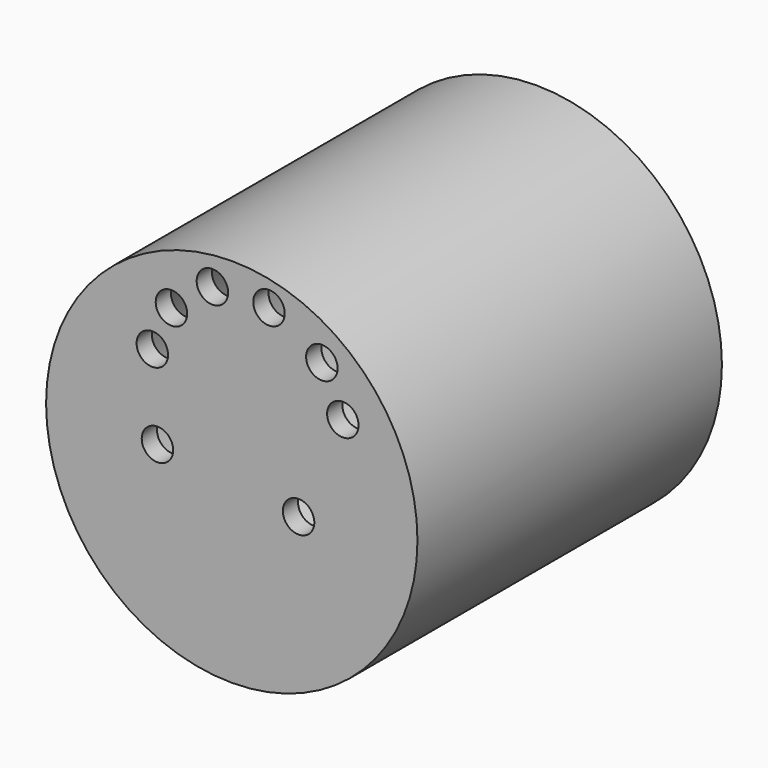
from build123d import *

# Parameters (mm, degrees)
F0_R     = 24.7867182939
F1_DEPTH = 50.8
F2_T     = -2.54
F7_D     = 4.2


# Not quite as in the source:
# - a feature of the source that left no trace in its solid (it failed there, or was rolled back) is left out


with BuildPart() as f1:
    # F0 (on Front) → F1 (new body)
    with BuildSketch(Plane.XZ):
        Circle(F0_R)
    extrude(amount=F1_DEPTH)

    # F2
    f2_openings = [f1.faces().sort_by_distance(p)[0] for p in [
        (0, 0, 0),
    ]]
    offset(amount=F2_T, openings=f2_openings)

    # F7 (through all)
    with Locations(Plane(origin=(0, 0, 0), x_dir=(1, 0, 0), z_dir=(0, 1, 0))):
        with Locations((8.9164366946, 2.3716597352), (14.8237738758, -10.9670488164), (12.0239807293, -16.7495105416), (4.9703707919, -20.9065452218), (-2.5862243492, -20.9065452218), (-8.0531220883, -16.6528206319), (-10.6035573408, -10.9806992114), (-9.9196853116, 0)):
            Hole(F7_D / 2)


solid = f1.part
